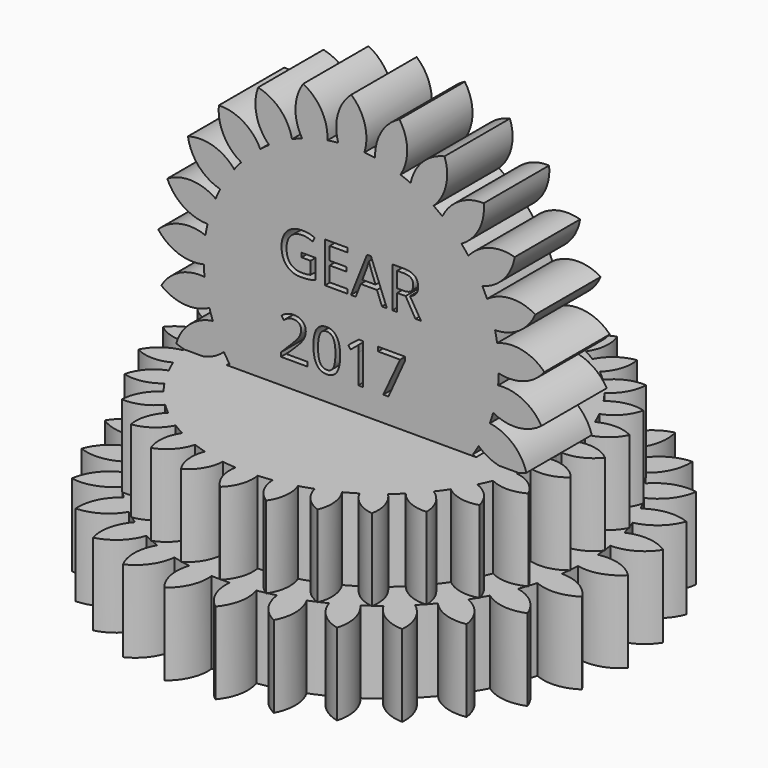
from build123d import *

# Parameters (mm, degrees)
F1_DEPTH     = 25.4
F3_DEPTH     = 25.4
F5_DEPTH     = 12.7
F6_TEXT_SIZE = 17.6388888889
F7_DEPTH     = 88.1229748473


# Not quite as in the source:
# - Text() gives the source's letters only with a copy of the font that has no kerning and outlines rounded to 1/6400 em; it was checked with that copy


with BuildPart() as f1:
    # F0 (on Top) → F1 (new body)
    with BuildSketch(Plane.XY):
        with BuildLine():
            ThreePointArc((63.3843742532, -3.8302872647), (63.4710869809, -1.9160160388), (63.5, 0))
            ThreePointArc((63.5, 0), (63.4710869809, 1.9160160388), (63.3843742532, 3.8302872647))
            ThreePointArc((63.3843742532, 3.8302872647), (63.1521403559, 6.6375574175), (62.7956351013, 9.4317661243))
            ThreePointArc((62.7956351013, 9.4317661243), (62.1123726466, 13.2023923669), (61.2029120983, 16.9249387205))
            ThreePointArc((61.2029120983, 16.9249387205), (60.3920887847, 19.6225791428), (59.4624253686, 22.2816060751))
            ThreePointArc((59.4624253686, 22.2816060751), (58.0101365603, 25.8277768353), (56.3465890005, 29.2798891393))
            ThreePointArc((56.3465890005, 29.2798891393), (54.9926131403, 31.75), (53.5304223149, 34.1576329213))
            ThreePointArc((53.5304223149, 34.1576329213), (51.3725791428, 37.3243635206), (49.0276495824, 40.3551679023))
            ThreePointArc((49.0276495824, 40.3551679023), (47.1896964178, 42.4897935038), (45.2588829386, 44.5408073024))
            ThreePointArc((45.2588829386, 44.5408073024), (42.4897935038, 47.1896964178), (39.5659666169, 49.6667321823))
            ThreePointArc((39.5659666169, 49.6667321823), (37.3243635206, 51.3725791428), (35.0093132016, 52.9773346739))
            ThreePointArc((35.0093132016, 52.9773346739), (31.75, 54.9926131403), (28.3750610516, 56.8076219386))
            ThreePointArc((28.3750610516, 56.8076219386), (25.8277768353, 58.0101365603), (23.2296684844, 59.0984983067))
            ThreePointArc((23.2296684844, 59.0984983067), (19.6225791428, 60.3920887847), (15.9440291597, 61.4657460229))
            ThreePointArc((15.9440291597, 61.4657460229), (13.2023923669, 62.1123726466), (10.4347757862, 62.6367739774))
            ThreePointArc((10.4347757862, 62.6367739774), (6.6375574175, 63.1521403559), (2.8161666856, 63.4375220607))
            ThreePointArc((2.8161666856, 63.4375220607), (0, 63.5), (-2.8161666856, 63.4375220607))
            ThreePointArc((-2.8161666856, 63.4375220607), (-6.6375574175, 63.1521403559), (-10.4347757862, 62.6367739774))
            ThreePointArc((-10.4347757862, 62.6367739774), (-13.2023923669, 62.1123726466), (-15.9440291597, 61.4657460229))
            ThreePointArc((-15.9440291597, 61.4657460229), (-19.6225791428, 60.3920887847), (-23.2296684844, 59.0984983067))
            ThreePointArc((-23.2296684844, 59.0984983067), (-25.8277768353, 58.0101365603), (-28.3750610516, 56.8076219386))
            ThreePointArc((-28.3750610516, 56.8076219386), (-31.75, 54.9926131403), (-35.0093132016, 52.9773346739))
            ThreePointArc((-35.0093132016, 52.9773346739), (-37.3243635206, 51.3725791428), (-39.5659666169, 49.6667321823))
            ThreePointArc((-39.5659666169, 49.6667321823), (-42.4897935038, 47.1896964178), (-45.2588829386, 44.5408073024))
            ThreePointArc((-45.2588829386, 44.5408073024), (-47.1896964178, 42.4897935038), (-49.0276495824, 40.3551679023))
            ThreePointArc((-49.0276495824, 40.3551679023), (-51.3725791428, 37.3243635206), (-53.5304223149, 34.1576329213))
            ThreePointArc((-53.5304223149, 34.1576329213), (-54.9926131403, 31.75), (-56.3465890005, 29.2798891393))
            ThreePointArc((-56.3465890005, 29.2798891393), (-58.0101365603, 25.8277768353), (-59.4624253686, 22.2816060751))
            ThreePointArc((-59.4624253686, 22.2816060751), (-60.3920887847, 19.6225791428), (-61.2029120983, 16.9249387205))
            ThreePointArc((-61.2029120983, 16.9249387205), (-62.1123726466, 13.2023923669), (-62.7956351013, 9.4317661243))
            ThreePointArc((-62.7956351013, 9.4317661243), (-63.1521403559, 6.6375574175), (-63.3843742532, 3.8302872647))
            ThreePointArc((-63.3843742532, 3.8302872647), (-63.5, 0), (-63.3843742532, -3.8302872647))
            ThreePointArc((-63.3843742532, -3.8302872647), (-63.1521403559, -6.6375574175), (-62.7956351013, -9.4317661243))
            ThreePointArc((-62.7956351013, -9.4317661243), (-62.1123726466, -13.2023923669), (-61.2029120983, -16.9249387205))
            ThreePointArc((-61.2029120983, -16.9249387205), (-60.3920887847, -19.6225791428), (-59.4624253686, -22.2816060751))
            ThreePointArc((-59.4624253686, -22.2816060751), (-58.0101365603, -25.8277768353), (-56.3465890005, -29.2798891393))
            ThreePointArc((-56.3465890005, -29.2798891393), (-54.9926131403, -31.75), (-53.5304223149, -34.1576329213))
            ThreePointArc((-53.5304223149, -34.1576329213), (-51.3725791428, -37.3243635206), (-49.0276495824, -40.3551679023))
            ThreePointArc((-49.0276495824, -40.3551679023), (-47.1896964178, -42.4897935038), (-45.2588829386, -44.5408073024))
            ThreePointArc((-45.2588829386, -44.5408073024), (-42.4897935038, -47.1896964178), (-39.5659666169, -49.6667321823))
            ThreePointArc((-39.5659666169, -49.6667321823), (-37.3243635206, -51.3725791428), (-35.0093132016, -52.9773346739))
            ThreePointArc((-35.0093132016, -52.9773346739), (-31.75, -54.9926131403), (-28.3750610516, -56.8076219386))
            ThreePointArc((-28.3750610516, -56.8076219386), (-25.8277768353, -58.0101365603), (-23.2296684844, -59.0984983067))
            ThreePointArc((-23.2296684844, -59.0984983067), (-19.6225791428, -60.3920887847), (-15.9440291597, -61.4657460229))
            ThreePointArc((-15.9440291597, -61.4657460229), (-13.2023923669, -62.1123726466), (-10.4347757862, -62.6367739774))
            ThreePointArc((-10.4347757862, -62.6367739774), (-6.6375574175, -63.1521403559), (-2.8161666856, -63.4375220607))
            ThreePointArc((-2.8161666856, -63.4375220607), (0, -63.5), (2.8161666856, -63.4375220607))
            ThreePointArc((2.8161666856, -63.4375220607), (6.6375574175, -63.1521403559), (10.4347757862, -62.6367739774))
            ThreePointArc((10.4347757862, -62.6367739774), (13.2023923669, -62.1123726466), (15.9440291597, -61.4657460229))
            ThreePointArc((15.9440291597, -61.4657460229), (19.6225791428, -60.3920887847), (23.2296684844, -59.0984983067))
            ThreePointArc((23.2296684844, -59.0984983067), (25.8277768353, -58.0101365603), (28.3750610516, -56.8076219386))
            ThreePointArc((28.3750610516, -56.8076219386), (31.75, -54.9926131403), (35.0093132016, -52.9773346739))
            ThreePointArc((35.0093132016, -52.9773346739), (37.3243635206, -51.3725791428), (39.5659666169, -49.6667321823))
            ThreePointArc((39.5659666169, -49.6667321823), (42.4897935038, -47.1896964178), (45.2588829386, -44.5408073024))
            ThreePointArc((45.2588829386, -44.5408073024), (47.1896964178, -42.4897935038), (49.0276495824, -40.3551679023))
            ThreePointArc((49.0276495824, -40.3551679023), (51.3725791428, -37.3243635206), (53.5304223149, -34.1576329213))
            ThreePointArc((53.5304223149, -34.1576329213), (54.9926131403, -31.75), (56.3465890005, -29.2798891393))
            ThreePointArc((56.3465890005, -29.2798891393), (58.0101365603, -25.8277768353), (59.4624253686, -22.2816060751))
            ThreePointArc((59.4624253686, -22.2816060751), (60.3920887847, -19.6225791428), (61.2029120983, -16.9249387205))
            ThreePointArc((61.2029120983, -16.9249387205), (62.1123726466, -13.2023923669), (62.7956351013, -9.4317661243))
            ThreePointArc((62.7956351013, -9.4317661243), (63.1521403559, -6.6375574175), (63.3843742532, -3.8302872647))
        make_face()
        with BuildLine():
            ThreePointArc((63.3843742532, 3.8302872647), (63.4710869809, 1.9160160388), (63.5, 0))
            ThreePointArc((63.5, 0), (63.4710869809, -1.9160160388), (63.3843742532, -3.8302872647))
            ThreePointArc((63.3843742532, -3.8302872647), (70.1108387826, -3.5405557516), (75.83742017, 0))
            ThreePointArc((75.83742017, 0), (70.1108387826, 3.5405557516), (63.3843742532, 3.8302872647))
        make_face()
        with BuildLine():
            ThreePointArc((61.2029120983, 16.9249387205), (62.1123726466, 13.2023923669), (62.7956351013, 9.4317661243))
            ThreePointArc((62.7956351013, 9.4317661243), (69.3148716734, 11.1136769223), (74.1801905851, 15.7674862548))
            ThreePointArc((74.1801905851, 15.7674862548), (67.8426258079, 18.0400491496), (61.2029120983, 16.9249387205))
        make_face()
        with BuildLine():
            ThreePointArc((74.1801905851, -15.7674862548), (69.3148716734, -11.1136769223), (62.7956351013, -9.4317661243))
            ThreePointArc((62.7956351013, -9.4317661243), (62.1123726466, -13.2023923669), (61.2029120983, -16.9249387205))
            ThreePointArc((61.2029120983, -16.9249387205), (67.8426258079, -18.0400491496), (74.1801905851, -15.7674862548))
        make_face()
        with BuildLine():
            ThreePointArc((56.3465890005, 29.2798891393), (58.0101365603, 25.8277768353), (59.4624253686, 22.2816060751))
            ThreePointArc((59.4624253686, 22.2816060751), (65.4895120624, 25.2821885853), (69.2809307156, 30.8458576995))
            ThreePointArc((69.2809307156, 30.8458576995), (62.6093645404, 31.751105834), (56.3465890005, 29.2798891393))
        make_face()
        with BuildLine():
            ThreePointArc((69.2809307156, -30.8458576995), (65.4895120624, -25.2821885853), (59.4624253686, -22.2816060751))
            ThreePointArc((59.4624253686, -22.2816060751), (58.0101365603, -25.8277768353), (56.3465890005, -29.2798891393))
            ThreePointArc((56.3465890005, -29.2798891393), (62.6093645404, -31.751105834), (69.2809307156, -30.8458576995))
        make_face()
        with BuildLine():
            ThreePointArc((49.0276495824, 40.3551679023), (51.3725791428, 37.3243635206), (53.5304223149, 34.1576329213))
            ThreePointArc((53.5304223149, 34.1576329213), (58.8019465207, 38.3457472898), (61.3537617271, 44.5761171478))
            ThreePointArc((61.3537617271, 44.5761171478), (54.6397736094, 44.0744868348), (49.0276495824, 40.3551679023))
        make_face()
        with BuildLine():
            ThreePointArc((61.3537617271, -44.5761171478), (58.8019465207, -38.3457472898), (53.5304223149, -34.1576329213))
            ThreePointArc((53.5304223149, -34.1576329213), (51.3725791428, -37.3243635206), (49.0276495824, -40.3551679023))
            ThreePointArc((49.0276495824, -40.3551679023), (54.6397736094, -44.0744868348), (61.3537617271, -44.5761171478))
        make_face()
        with BuildLine():
            ThreePointArc((39.5659666169, 49.6667321823), (42.4897935038, 47.1896964178), (45.2588829386, 44.5408073024))
            ThreePointArc((45.2588829386, 44.5408073024), (49.544453753, 49.7334128343), (50.745138943, 56.3581863769))
            ThreePointArc((50.745138943, 56.3581863769), (44.2821623809, 54.4716012681), (39.5659666169, 49.6667321823))
        make_face()
        with BuildLine():
            ThreePointArc((50.745138943, -56.3581863769), (49.544453753, -49.7334128343), (45.2588829386, -44.5408073024))
            ThreePointArc((45.2588829386, -44.5408073024), (42.4897935038, -47.1896964178), (39.5659666169, -49.6667321823))
            ThreePointArc((39.5659666169, -49.6667321823), (44.2821623809, -54.4716012681), (50.745138943, -56.3581863769))
        make_face()
        with BuildLine():
            ThreePointArc((28.3750610516, 56.8076219386), (31.75, 54.9926131403), (35.0093132016, 52.9773346739))
            ThreePointArc((35.0093132016, 52.9773346739), (38.1216306157, 58.9474895906), (37.918710085, 65.6771324247))
            ThreePointArc((37.918710085, 65.6771324247), (31.989208167, 62.4880453422), (28.3750610516, 56.8076219386))
        make_face()
        with BuildLine():
            ThreePointArc((37.918710085, -65.6771324247), (38.1216306157, -58.9474895906), (35.0093132016, -52.9773346739))
            ThreePointArc((35.0093132016, -52.9773346739), (31.75, -54.9926131403), (28.3750610516, -56.8076219386))
            ThreePointArc((28.3750610516, -56.8076219386), (31.989208167, -62.4880453422), (37.918710085, -65.6771324247))
        make_face()
        with BuildLine():
            ThreePointArc((15.9440291597, 61.4657460229), (19.6225791428, 60.3920887847), (23.2296684844, 59.0984983067))
            ThreePointArc((23.2296684844, 59.0984983067), (25.0327092925, 65.5852781904), (23.4350516421, 72.1256726317))
            ThreePointArc((23.4350516421, 72.1256726317), (18.2981720549, 67.7734619839), (15.9440291597, 61.4657460229))
        make_face()
        with BuildLine():
            ThreePointArc((23.4350516421, -72.1256726317), (25.0327092925, -65.5852781904), (23.2296684844, -59.0984983067))
            ThreePointArc((23.2296684844, -59.0984983067), (19.6225791428, -60.3920887847), (15.9440291597, -61.4657460229))
            ThreePointArc((15.9440291597, -61.4657460229), (18.2981720549, -67.7734619839), (23.4350516421, -72.1256726317))
        make_face()
        with BuildLine():
            ThreePointArc((2.8161666856, 63.4375220607), (6.6375574175, 63.1521403559), (10.4347757862, 62.6367739774))
            ThreePointArc((10.4347757862, 62.6367739774), (10.849738453, 69.3566754201), (7.9271689885, 75.4219748473))
            ThreePointArc((7.9271689885, 75.4219748473), (3.8074180197, 70.0968531238), (2.8161666856, 63.4375220607))
        make_face()
        with BuildLine():
            ThreePointArc((7.9271689885, -75.4219748473), (10.849738453, -69.3566754201), (10.4347757862, -62.6367739774))
            ThreePointArc((10.4347757862, -62.6367739774), (6.6375574175, -63.1521403559), (2.8161666856, -63.4375220607))
            ThreePointArc((2.8161666856, -63.4375220607), (3.8074180197, -70.0968531238), (7.9271689885, -75.4219748473))
        make_face()
        with BuildLine():
            ThreePointArc((-10.4347757862, 62.6367739774), (-6.6375574175, 63.1521403559), (-2.8161666856, 63.4375220607))
            ThreePointArc((-2.8161666856, 63.4375220607), (-3.8074180197, 70.0968531238), (-7.9271689885, 75.4219748473))
            ThreePointArc((-7.9271689885, 75.4219748473), (-10.849738453, 69.3566754201), (-10.4347757862, 62.6367739774))
        make_face()
        with BuildLine():
            ThreePointArc((-7.9271689885, -75.4219748473), (-3.8074180197, -70.0968531238), (-2.8161666856, -63.4375220607))
            ThreePointArc((-2.8161666856, -63.4375220607), (-6.6375574175, -63.1521403559), (-10.4347757862, -62.6367739774))
            ThreePointArc((-10.4347757862, -62.6367739774), (-10.849738453, -69.3566754201), (-7.9271689885, -75.4219748473))
        make_face()
        with BuildLine():
            ThreePointArc((-23.2296684844, 59.0984983067), (-19.6225791428, 60.3920887847), (-15.9440291597, 61.4657460229))
            ThreePointArc((-15.9440291597, 61.4657460229), (-18.2981720549, 67.7734619839), (-23.4350516421, 72.1256726317))
            ThreePointArc((-23.4350516421, 72.1256726317), (-25.0327092925, 65.5852781904), (-23.2296684844, 59.0984983067))
        make_face()
        with BuildLine():
            ThreePointArc((-23.4350516421, -72.1256726317), (-18.2981720549, -67.7734619839), (-15.9440291597, -61.4657460229))
            ThreePointArc((-15.9440291597, -61.4657460229), (-19.6225791428, -60.3920887847), (-23.2296684844, -59.0984983067))
            ThreePointArc((-23.2296684844, -59.0984983067), (-25.0327092925, -65.5852781904), (-23.4350516421, -72.1256726317))
        make_face()
        with BuildLine():
            ThreePointArc((-35.0093132016, 52.9773346739), (-31.75, 54.9926131403), (-28.3750610516, 56.8076219386))
            ThreePointArc((-28.3750610516, 56.8076219386), (-31.989208167, 62.4880453422), (-37.918710085, 65.6771324247))
            ThreePointArc((-37.918710085, 65.6771324247), (-38.1216306157, 58.9474895906), (-35.0093132016, 52.9773346739))
        make_face()
        with BuildLine():
            ThreePointArc((-37.918710085, -65.6771324247), (-31.989208167, -62.4880453422), (-28.3750610516, -56.8076219386))
            ThreePointArc((-28.3750610516, -56.8076219386), (-31.75, -54.9926131403), (-35.0093132016, -52.9773346739))
            ThreePointArc((-35.0093132016, -52.9773346739), (-38.1216306157, -58.9474895906), (-37.918710085, -65.6771324247))
        make_face()
        with BuildLine():
            ThreePointArc((-45.2588829386, 44.5408073024), (-42.4897935038, 47.1896964178), (-39.5659666169, 49.6667321823))
            ThreePointArc((-39.5659666169, 49.6667321823), (-44.2821623809, 54.4716012681), (-50.745138943, 56.3581863769))
            ThreePointArc((-50.745138943, 56.3581863769), (-49.544453753, 49.7334128343), (-45.2588829386, 44.5408073024))
        make_face()
        with BuildLine():
            ThreePointArc((-50.745138943, -56.3581863769), (-44.2821623809, -54.4716012681), (-39.5659666169, -49.6667321823))
            ThreePointArc((-39.5659666169, -49.6667321823), (-42.4897935038, -47.1896964178), (-45.2588829386, -44.5408073024))
            ThreePointArc((-45.2588829386, -44.5408073024), (-49.544453753, -49.7334128343), (-50.745138943, -56.3581863769))
        make_face()
        with BuildLine():
            ThreePointArc((-53.5304223149, 34.1576329213), (-51.3725791428, 37.3243635206), (-49.0276495824, 40.3551679023))
            ThreePointArc((-49.0276495824, 40.3551679023), (-54.6397736094, 44.0744868348), (-61.3537617271, 44.5761171478))
            ThreePointArc((-61.3537617271, 44.5761171478), (-58.8019465207, 38.3457472898), (-53.5304223149, 34.1576329213))
        make_face()
        with BuildLine():
            ThreePointArc((-61.3537617271, -44.5761171478), (-54.6397736094, -44.0744868348), (-49.0276495824, -40.3551679023))
            ThreePointArc((-49.0276495824, -40.3551679023), (-51.3725791428, -37.3243635206), (-53.5304223149, -34.1576329213))
            ThreePointArc((-53.5304223149, -34.1576329213), (-58.8019465207, -38.3457472898), (-61.3537617271, -44.5761171478))
        make_face()
        with BuildLine():
            ThreePointArc((-59.4624253686, 22.2816060751), (-58.0101365603, 25.8277768353), (-56.3465890005, 29.2798891393))
            ThreePointArc((-56.3465890005, 29.2798891393), (-62.6093645404, 31.751105834), (-69.2809307156, 30.8458576995))
            ThreePointArc((-69.2809307156, 30.8458576995), (-65.4895120624, 25.2821885853), (-59.4624253686, 22.2816060751))
        make_face()
        with BuildLine():
            ThreePointArc((-69.2809307156, -30.8458576995), (-62.6093645404, -31.751105834), (-56.3465890005, -29.2798891393))
            ThreePointArc((-56.3465890005, -29.2798891393), (-58.0101365603, -25.8277768353), (-59.4624253686, -22.2816060751))
            ThreePointArc((-59.4624253686, -22.2816060751), (-65.4895120624, -25.2821885853), (-69.2809307156, -30.8458576995))
        make_face()
        with BuildLine():
            ThreePointArc((-62.7956351013, 9.4317661243), (-62.1123726466, 13.2023923669), (-61.2029120983, 16.9249387205))
            ThreePointArc((-61.2029120983, 16.9249387205), (-67.8426258079, 18.0400491496), (-74.1801905851, 15.7674862548))
            ThreePointArc((-74.1801905851, 15.7674862548), (-69.3148716734, 11.1136769223), (-62.7956351013, 9.4317661243))
        make_face()
        with BuildLine():
            ThreePointArc((-74.1801905851, -15.7674862548), (-67.8426258079, -18.0400491496), (-61.2029120983, -16.9249387205))
            ThreePointArc((-61.2029120983, -16.9249387205), (-62.1123726466, -13.2023923669), (-62.7956351013, -9.4317661243))
            ThreePointArc((-62.7956351013, -9.4317661243), (-69.3148716734, -11.1136769223), (-74.1801905851, -15.7674862548))
        make_face()
        with BuildLine():
            ThreePointArc((-63.3843742532, -3.8302872647), (-63.9551391112, 0), (-63.3843742532, 3.8302872647))
            ThreePointArc((-63.3843742532, 3.8302872647), (-70.1108387826, 3.5405557516), (-75.83742017, 0))
            ThreePointArc((-75.83742017, 0), (-70.1108387826, -3.5405557516), (-63.3843742532, -3.8302872647))
        make_face()
        with BuildLine():
            ThreePointArc((-63.3843742532, -3.8302872647), (-63.5, 0), (-63.3843742532, 3.8302872647))
            ThreePointArc((-63.3843742532, 3.8302872647), (-63.9551391112, 0), (-63.3843742532, -3.8302872647))
        make_face()
    extrude(amount=F1_DEPTH)

    # F2 (on face) → F3 (join)
    with BuildSketch(Plane.XY.offset(25.4)):
        with BuildLine():
            ThreePointArc((53.4574080141, -2.1584102312), (53.4900742973, -1.0794248349), (53.5009645362, 0))
            ThreePointArc((53.5009645362, 0), (53.4900742973, 1.0794248349), (53.4574080141, 2.1584102312))
            ThreePointArc((53.4574080141, 2.1584102312), (53.2078806546, 5.5923736063), (52.7379941111, 9.0031762979))
            ThreePointArc((52.7379941111, 9.0031762979), (52.3318400981, 11.1234759971), (51.8404766698, 13.225663876))
            ThreePointArc((51.8404766698, 13.225663876), (50.8824409503, 16.5327072572), (49.7136768004, 19.7712808207))
            ThreePointArc((49.7136768004, 19.7712808207), (48.8755631316, 21.7608027168), (47.9578677368, 23.7148925456))
            ThreePointArc((47.9578677368, 23.7148925456), (46.3331944154, 26.7504822681), (44.5166332609, 29.6752854986))
            ThreePointArc((44.5166332609, 29.6752854986), (43.2831895253, 31.4470779378), (41.9792698563, 33.1676666143))
            ThreePointArc((41.9792698563, 33.1676666143), (39.7589649532, 35.7991328409), (37.3739992334, 38.2823378023))
            ThreePointArc((37.3739992334, 38.2823378023), (35.7991328409, 39.7589649532), (34.1659764442, 41.1708544959))
            ThreePointArc((34.1659764442, 41.1708544959), (31.4470779378, 43.2831895253), (28.5979420991, 45.216268245))
            ThreePointArc((28.5979420991, 45.216268245), (26.7504822681, 46.3331944154), (24.859465915, 47.3746784763))
            ThreePointArc((24.859465915, 47.3746784763), (21.7608027168, 48.8755631316), (18.5720176668, 50.1740307937))
            ThreePointArc((18.5720176668, 50.1740307937), (16.5327072572, 50.8824409503), (14.4664774363, 51.5080016783))
            ThreePointArc((14.4664774363, 51.5080016783), (11.1234759971, 52.3318400981), (7.7344069441, 52.9389474351))
            ThreePointArc((7.7344069441, 52.9389474351), (5.5923736063, 53.2078806546), (3.4412344758, 53.3901780442))
            ThreePointArc((3.4412344758, 53.3901780442), (0, 53.5009645362), (-3.4412344758, 53.3901780442))
            ThreePointArc((-3.4412344758, 53.3901780442), (-5.5923736063, 53.2078806546), (-7.7344069441, 52.9389474351))
            ThreePointArc((-7.7344069441, 52.9389474351), (-11.1234759971, 52.3318400981), (-14.4664774363, 51.5080016783))
            ThreePointArc((-14.4664774363, 51.5080016783), (-16.5327072572, 50.8824409503), (-18.5720176668, 50.1740307937))
            ThreePointArc((-18.5720176668, 50.1740307937), (-21.7608027168, 48.8755631316), (-24.859465915, 47.3746784763))
            ThreePointArc((-24.859465915, 47.3746784763), (-26.7504822681, 46.3331944154), (-28.5979420991, 45.216268245))
            ThreePointArc((-28.5979420991, 45.216268245), (-31.4470779378, 43.2831895253), (-34.1659764442, 41.1708544959))
            ThreePointArc((-34.1659764442, 41.1708544959), (-35.7991328409, 39.7589649532), (-37.3739992334, 38.2823378023))
            ThreePointArc((-37.3739992334, 38.2823378023), (-39.7589649532, 35.7991328409), (-41.9792698563, 33.1676666143))
            ThreePointArc((-41.9792698563, 33.1676666143), (-43.2831895253, 31.4470779378), (-44.5166332609, 29.6752854986))
            ThreePointArc((-44.5166332609, 29.6752854986), (-46.3331944154, 26.7504822681), (-47.9578677368, 23.7148925456))
            ThreePointArc((-47.9578677368, 23.7148925456), (-48.8755631316, 21.7608027168), (-49.7136768004, 19.7712808207))
            ThreePointArc((-49.7136768004, 19.7712808207), (-50.8824409503, 16.5327072572), (-51.8404766698, 13.225663876))
            ThreePointArc((-51.8404766698, 13.225663876), (-52.3318400981, 11.1234759971), (-52.7379941111, 9.0031762979))
            ThreePointArc((-52.7379941111, 9.0031762979), (-52.9098679132, 7.2911544424), (-53.0870626478, 5.5796751221))
            ThreePointArc((-53.0870626478, 5.5796751221), (-53.2695766026, 3.8687548744), (-53.4574080141, 2.1584102312))
            ThreePointArc((-53.4574080141, 2.1584102312), (-53.5009645362, 0), (-53.4574080141, -2.1584102312))
            ThreePointArc((-53.4574080141, -2.1584102312), (-53.2078806546, -5.5923736063), (-52.7379941111, -9.0031762979))
            ThreePointArc((-52.7379941111, -9.0031762979), (-52.3318400981, -11.1234759971), (-51.8404766698, -13.225663876))
            ThreePointArc((-51.8404766698, -13.225663876), (-50.8824409503, -16.5327072572), (-49.7136768004, -19.7712808207))
            ThreePointArc((-49.7136768004, -19.7712808207), (-48.8755631316, -21.7608027168), (-47.9578677368, -23.7148925456))
            ThreePointArc((-47.9578677368, -23.7148925456), (-46.3331944154, -26.7504822681), (-44.5166332609, -29.6752854986))
            ThreePointArc((-44.5166332609, -29.6752854986), (-43.2831895253, -31.4470779378), (-41.9792698563, -33.1676666143))
            ThreePointArc((-41.9792698563, -33.1676666143), (-39.7589649532, -35.7991328409), (-37.3739992334, -38.2823378023))
            ThreePointArc((-37.3739992334, -38.2823378023), (-35.7991328409, -39.7589649532), (-34.1659764442, -41.1708544959))
            ThreePointArc((-34.1659764442, -41.1708544959), (-31.4470779378, -43.2831895253), (-28.5979420991, -45.216268245))
            ThreePointArc((-28.5979420991, -45.216268245), (-26.7504822681, -46.3331944154), (-24.859465915, -47.3746784763))
            ThreePointArc((-24.859465915, -47.3746784763), (-21.7608027168, -48.8755631316), (-18.5720176668, -50.1740307937))
            ThreePointArc((-18.5720176668, -50.1740307937), (-16.5327072572, -50.8824409503), (-14.4664774363, -51.5080016783))
            ThreePointArc((-14.4664774363, -51.5080016783), (-11.1234759971, -52.3318400981), (-7.7344069441, -52.9389474351))
            ThreePointArc((-7.7344069441, -52.9389474351), (-5.5923736063, -53.2078806546), (-3.4412344758, -53.3901780442))
            ThreePointArc((-3.4412344758, -53.3901780442), (0, -53.5009645362), (3.4412344758, -53.3901780442))
            ThreePointArc((3.4412344758, -53.3901780442), (5.5923736063, -53.2078806546), (7.7344069441, -52.9389474351))
            ThreePointArc((7.7344069441, -52.9389474351), (11.1234759971, -52.3318400981), (14.4664774363, -51.5080016783))
            ThreePointArc((14.4664774363, -51.5080016783), (16.5327072572, -50.8824409503), (18.5720176668, -50.1740307937))
            ThreePointArc((18.5720176668, -50.1740307937), (21.7608027168, -48.8755631316), (24.859465915, -47.3746784763))
            ThreePointArc((24.859465915, -47.3746784763), (26.7504822681, -46.3331944154), (28.5979420991, -45.216268245))
            ThreePointArc((28.5979420991, -45.216268245), (31.4470779378, -43.2831895253), (34.1659764442, -41.1708544959))
            ThreePointArc((34.1659764442, -41.1708544959), (35.7991328409, -39.7589649532), (37.3739992334, -38.2823378023))
            ThreePointArc((37.3739992334, -38.2823378023), (39.7589649532, -35.7991328409), (41.9792698563, -33.1676666143))
            ThreePointArc((41.9792698563, -33.1676666143), (43.2831895253, -31.4470779378), (44.5166332609, -29.6752854986))
            ThreePointArc((44.5166332609, -29.6752854986), (46.3331944154, -26.7504822681), (47.9578677368, -23.7148925456))
            ThreePointArc((47.9578677368, -23.7148925456), (48.8755631316, -21.7608027168), (49.7136768004, -19.7712808207))
            ThreePointArc((49.7136768004, -19.7712808207), (50.8824409503, -16.5327072572), (51.8404766698, -13.225663876))
            ThreePointArc((51.8404766698, -13.225663876), (52.3318400981, -11.1234759971), (52.7379941111, -9.0031762979))
            ThreePointArc((52.7379941111, -9.0031762979), (53.2078806546, -5.5923736063), (53.4574080141, -2.1584102312))
        make_face()
        with BuildLine():
            ThreePointArc((52.7379941111, 9.0031762979), (53.2078806546, 5.5923736063), (53.4574080141, 2.1584102312))
            ThreePointArc((53.4574080141, 2.1584102312), (58.9731507298, 3.1661170371), (63.3590941473, 6.6593091375))
            ThreePointArc((63.3590941473, 6.6593091375), (58.3427186405, 9.1642776976), (52.7379941111, 9.0031762979))
        make_face()
        with BuildLine():
            ThreePointArc((63.3590941473, -6.6593091375), (58.9731507298, -3.1661170371), (53.4574080141, -2.1584102312))
            ThreePointArc((53.4574080141, -2.1584102312), (53.2078806546, -5.5923736063), (52.7379941111, -9.0031762979))
            ThreePointArc((52.7379941111, -9.0031762979), (58.3427186405, -9.1642776976), (63.3590941473, -6.6593091375))
        make_face()
        with BuildLine():
            ThreePointArc((49.7136768004, 19.7712808207), (50.8824409503, 16.5327072572), (51.8404766698, 13.225663876))
            ThreePointArc((51.8404766698, 13.225663876), (57.0261731475, 15.3581372645), (60.5899977024, 19.6868836482))
            ThreePointArc((60.5899977024, 19.6868836482), (55.1624297873, 21.0941495218), (49.7136768004, 19.7712808207))
        make_face()
        with BuildLine():
            ThreePointArc((60.5899977024, -19.6868836482), (57.0261731475, -15.3581372645), (51.8404766698, -13.225663876))
            ThreePointArc((51.8404766698, -13.225663876), (50.8824409503, -16.5327072572), (49.7136768004, -19.7712808207))
            ThreePointArc((49.7136768004, -19.7712808207), (55.1624297873, -21.0941495218), (60.5899977024, -19.6868836482))
        make_face()
        with BuildLine():
            ThreePointArc((44.5166332609, 29.6752854986), (46.3331944154, 26.7504822681), (47.9578677368, 23.7148925456))
            ThreePointArc((47.9578677368, 23.7148925456), (52.5868781568, 26.878933197), (55.1728276148, 31.8540468754))
            ThreePointArc((55.1728276148, 31.8540468754), (49.5712780536, 32.102105791), (44.5166332609, 29.6752854986))
        make_face()
        with BuildLine():
            ThreePointArc((55.1728276148, -31.8540468754), (52.5868781568, -26.878933197), (47.9578677368, -23.7148925456))
            ThreePointArc((47.9578677368, -23.7148925456), (46.3331944154, -26.7504822681), (44.5166332609, -29.6752854986))
            ThreePointArc((44.5166332609, -29.6752854986), (49.5712780536, -32.102105791), (55.1728276148, -31.8540468754))
        make_face()
        with BuildLine():
            ThreePointArc((37.3739992334, 38.2823378023), (39.7589649532, 35.7991328409), (41.9792698563, 33.1676666143))
            ThreePointArc((41.9792698563, 33.1676666143), (45.8492842508, 37.2249907694), (47.3443402119, 42.6290354014))
            ThreePointArc((47.3443402119, 42.6290354014), (41.8136235997, 41.7070459941), (37.3739992334, 38.2823378023))
        make_face()
        with BuildLine():
            ThreePointArc((47.3443402119, -42.6290354014), (45.8492842508, -37.2249907694), (41.9792698563, -33.1676666143))
            ThreePointArc((41.9792698563, -33.1676666143), (39.7589649532, -35.7991328409), (37.3739992334, -38.2823378023))
            ThreePointArc((37.3739992334, -38.2823378023), (41.8136235997, -41.7070459941), (47.3443402119, -42.6290354014))
        make_face()
        with BuildLine():
            ThreePointArc((28.5979420991, 45.216268245), (31.4470779378, 43.2831895253), (34.1659764442, 41.1708544959))
            ThreePointArc((34.1659764442, 41.1708544959), (37.1078566137, 45.9441376197), (37.4466779584, 51.5409305236))
            ThreePointArc((37.4466779584, 51.5409305236), (32.2285131503, 49.4891881546), (28.5979420991, 45.216268245))
        make_face()
        with BuildLine():
            ThreePointArc((37.4466779584, -51.5409305236), (37.1078566137, -45.9441376197), (34.1659764442, -41.1708544959))
            ThreePointArc((34.1659764442, -41.1708544959), (31.4470779378, -43.2831895253), (28.5979420991, -45.216268245))
            ThreePointArc((28.5979420991, -45.216268245), (32.2285131503, -49.4891881546), (37.4466779584, -51.5409305236))
        make_face()
        with BuildLine():
            ThreePointArc((18.5720176668, 50.1740307937), (21.7608027168, 48.8755631316), (24.859465915, 47.3746784763))
            ThreePointArc((24.859465915, 47.3746784763), (26.7446375794, 52.6553051917), (25.9124161889, 58.2002396611))
            ThreePointArc((25.9124161889, 58.2002396611), (21.2348620268, 55.1084153173), (18.5720176668, 50.1740307937))
        make_face()
        with BuildLine():
            ThreePointArc((25.9124161889, -58.2002396611), (26.7446375794, -52.6553051917), (24.859465915, -47.3746784763))
            ThreePointArc((24.859465915, -47.3746784763), (21.7608027168, -48.8755631316), (18.5720176668, -50.1740307937))
            ThreePointArc((18.5720176668, -50.1740307937), (21.2348620268, -55.1084153173), (25.9124161889, -58.2002396611))
        make_face()
        with BuildLine():
            ThreePointArc((7.7344069441, 52.9389474351), (11.1234759971, 52.3318400981), (14.4664774363, 51.5080016783))
            ThreePointArc((14.4664774363, 51.5080016783), (15.2125495479, 57.0651832586), (13.2456574905, 62.3159190496))
            ThreePointArc((13.2456574905, 62.3159190496), (9.3131455365, 58.3191402912), (7.7344069441, 52.9389474351))
        make_face()
        with BuildLine():
            ThreePointArc((13.2456574905, -62.3159190496), (15.2125495479, -57.0651832586), (14.4664774363, -51.5080016783))
            ThreePointArc((14.4664774363, -51.5080016783), (11.1234759971, -52.3318400981), (7.7344069441, -52.9389474351))
            ThreePointArc((7.7344069441, -52.9389474351), (9.3131455365, -58.3191402912), (13.2456574905, -62.3159190496))
        make_face()
        with BuildLine():
            ThreePointArc((-3.4412344758, 53.3901780442), (0, 53.5009645362), (3.4412344758, 53.3901780442))
            ThreePointArc((3.4412344758, 53.3901780442), (3.0156001031, 58.981038988), (0, 63.7080937508))
            ThreePointArc((0, 63.7080937508), (-3.0156001031, 58.981038988), (-3.4412344758, 53.3901780442))
        make_face()
        with BuildLine():
            ThreePointArc((0, -63.7080937508), (3.0156001031, -58.981038988), (3.4412344758, -53.3901780442))
            ThreePointArc((3.4412344758, -53.3901780442), (0, -53.5009645362), (-3.4412344758, -53.3901780442))
            ThreePointArc((-3.4412344758, -53.3901780442), (-3.0156001031, -58.981038988), (0, -63.7080937508))
        make_face()
        with BuildLine():
            ThreePointArc((-14.4664774363, 51.5080016783), (-11.1234759971, 52.3318400981), (-7.7344069441, 52.9389474351))
            ThreePointArc((-7.7344069441, 52.9389474351), (-9.3131455365, 58.3191402912), (-13.2456574905, 62.3159190496))
            ThreePointArc((-13.2456574905, 62.3159190496), (-15.2125495479, 57.0651832586), (-14.4664774363, 51.5080016783))
        make_face()
        with BuildLine():
            ThreePointArc((-13.2456574905, -62.3159190496), (-9.3131455365, -58.3191402912), (-7.7344069441, -52.9389474351))
            ThreePointArc((-7.7344069441, -52.9389474351), (-11.1234759971, -52.3318400981), (-14.4664774363, -51.5080016783))
            ThreePointArc((-14.4664774363, -51.5080016783), (-15.2125495479, -57.0651832586), (-13.2456574905, -62.3159190496))
        make_face()
        with BuildLine():
            ThreePointArc((-24.859465915, 47.3746784763), (-21.7608027168, 48.8755631316), (-18.5720176668, 50.1740307937))
            ThreePointArc((-18.5720176668, 50.1740307937), (-21.2348620268, 55.1084153173), (-25.9124161889, 58.2002396611))
            ThreePointArc((-25.9124161889, 58.2002396611), (-26.7446375794, 52.6553051917), (-24.859465915, 47.3746784763))
        make_face()
        with BuildLine():
            ThreePointArc((-25.9124161889, -58.2002396611), (-21.2348620268, -55.1084153173), (-18.5720176668, -50.1740307937))
            ThreePointArc((-18.5720176668, -50.1740307937), (-21.7608027168, -48.8755631316), (-24.859465915, -47.3746784763))
            ThreePointArc((-24.859465915, -47.3746784763), (-26.7446375794, -52.6553051917), (-25.9124161889, -58.2002396611))
        make_face()
        with BuildLine():
            ThreePointArc((-34.1659764442, 41.1708544959), (-31.4470779378, 43.2831895253), (-28.5979420991, 45.216268245))
            ThreePointArc((-28.5979420991, 45.216268245), (-32.2285131503, 49.4891881546), (-37.4466779584, 51.5409305236))
            ThreePointArc((-37.4466779584, 51.5409305236), (-37.1078566137, 45.9441376197), (-34.1659764442, 41.1708544959))
        make_face()
        with BuildLine():
            ThreePointArc((-37.4466779584, -51.5409305236), (-32.2285131503, -49.4891881546), (-28.5979420991, -45.216268245))
            ThreePointArc((-28.5979420991, -45.216268245), (-31.4470779378, -43.2831895253), (-34.1659764442, -41.1708544959))
            ThreePointArc((-34.1659764442, -41.1708544959), (-37.1078566137, -45.9441376197), (-37.4466779584, -51.5409305236))
        make_face()
        with BuildLine():
            ThreePointArc((-41.9792698563, 33.1676666143), (-39.7589649532, 35.7991328409), (-37.3739992334, 38.2823378023))
            ThreePointArc((-37.3739992334, 38.2823378023), (-41.8136235997, 41.7070459941), (-47.3443402119, 42.6290354014))
            ThreePointArc((-47.3443402119, 42.6290354014), (-45.8492842508, 37.2249907694), (-41.9792698563, 33.1676666143))
        make_face()
        with BuildLine():
            ThreePointArc((-47.3443402119, -42.6290354014), (-41.8136235997, -41.7070459941), (-37.3739992334, -38.2823378023))
            ThreePointArc((-37.3739992334, -38.2823378023), (-39.7589649532, -35.7991328409), (-41.9792698563, -33.1676666143))
            ThreePointArc((-41.9792698563, -33.1676666143), (-45.8492842508, -37.2249907694), (-47.3443402119, -42.6290354014))
        make_face()
        with BuildLine():
            ThreePointArc((-47.9578677368, 23.7148925456), (-46.3331944154, 26.7504822681), (-44.5166332609, 29.6752854986))
            ThreePointArc((-44.5166332609, 29.6752854986), (-49.5712780536, 32.102105791), (-55.1728276148, 31.8540468754))
            ThreePointArc((-55.1728276148, 31.8540468754), (-52.5868781568, 26.878933197), (-47.9578677368, 23.7148925456))
        make_face()
        with BuildLine():
            ThreePointArc((-55.1728276148, -31.8540468754), (-49.5712780536, -32.102105791), (-44.5166332609, -29.6752854986))
            ThreePointArc((-44.5166332609, -29.6752854986), (-46.3331944154, -26.7504822681), (-47.9578677368, -23.7148925456))
            ThreePointArc((-47.9578677368, -23.7148925456), (-52.5868781568, -26.878933197), (-55.1728276148, -31.8540468754))
        make_face()
        with BuildLine():
            ThreePointArc((-51.8404766698, 13.225663876), (-50.8824409503, 16.5327072572), (-49.7136768004, 19.7712808207))
            ThreePointArc((-49.7136768004, 19.7712808207), (-55.1624297873, 21.0941495218), (-60.5899977024, 19.6868836482))
            ThreePointArc((-60.5899977024, 19.6868836482), (-57.0261731475, 15.3581372645), (-51.8404766698, 13.225663876))
        make_face()
        with BuildLine():
            ThreePointArc((-60.5899977024, -19.6868836482), (-55.1624297873, -21.0941495218), (-49.7136768004, -19.7712808207))
            ThreePointArc((-49.7136768004, -19.7712808207), (-50.8824409503, -16.5327072572), (-51.8404766698, -13.225663876))
            ThreePointArc((-51.8404766698, -13.225663876), (-57.0261731475, -15.3581372645), (-60.5899977024, -19.6868836482))
        make_face()
        with BuildLine():
            ThreePointArc((-53.0870626478, 5.5796751221), (-52.9098679132, 7.2911544424), (-52.7379941111, 9.0031762979))
            ThreePointArc((-52.7379941111, 9.0031762979), (-53.0003819676, 7.3015558337), (-53.2078806546, 5.5923736063))
            Line((-53.2078806546, 5.5923736063), (-53.0870626478, 5.5796751221))
        make_face()
        with BuildLine():
            ThreePointArc((-53.2078806546, 5.5923736063), (-53.0003819676, 7.3015558337), (-52.7379941111, 9.0031762979))
            ThreePointArc((-52.7379941111, 9.0031762979), (-58.3427186405, 9.1642776976), (-63.3590941473, 6.6593091375))
            ThreePointArc((-63.3590941473, 6.6593091375), (-58.9731507298, 3.1661170371), (-53.4574080141, 2.1584102312))
            ThreePointArc((-53.4574080141, 2.1584102312), (-53.3602752786, 3.8773997085), (-53.2078806546, 5.5923736063))
        make_face()
        with BuildLine():
            ThreePointArc((-63.3590941473, -6.6593091375), (-58.3427186405, -9.1642776976), (-52.7379941111, -9.0031762979))
            ThreePointArc((-52.7379941111, -9.0031762979), (-53.2078806546, -5.5923736063), (-53.4574080141, -2.1584102312))
            ThreePointArc((-53.4574080141, -2.1584102312), (-58.9731507298, -3.1661170371), (-63.3590941473, -6.6593091375))
        make_face()
        with BuildLine():
            Line((-53.0870626478, 5.5796751221), (-53.2078806546, 5.5923736063))
            ThreePointArc((-53.2078806546, 5.5923736063), (-53.3602752786, 3.8773997085), (-53.4574080141, 2.1584102312))
            ThreePointArc((-53.4574080141, 2.1584102312), (-53.2695766026, 3.8687548744), (-53.0870626478, 5.5796751221))
        make_face()
    extrude(amount=F3_DEPTH)

    # F4 (on Front) → F5 (join, symmetric)
    with BuildSketch(Plane.XZ):
        with BuildLine():
            ThreePointArc((45.8317549389, 76.044509612), (45.8433671556, 76.640169339), (45.8472381123, 77.2359296679))
            ThreePointArc((45.8472381123, 77.2359296679), (45.7154976418, 80.7090432407), (45.3210333338, 84.1621970673))
            ThreePointArc((45.3210333338, 84.1621970673), (45.0351574789, 85.8268454156), (44.6881601981, 87.4798342282))
            ThreePointArc((44.6881601981, 87.4798342282), (43.6033145609, 91.4035053898), (42.174697074, 95.2154783064))
            ThreePointArc((42.174697074, 95.2154783064), (41.4838213249, 96.7567342316), (40.7366440004, 98.2714966465))
            ThreePointArc((40.7366440004, 98.2714966465), (38.7101034454, 101.8021083243), (36.3783694894, 105.1390383804))
            ThreePointArc((36.3783694894, 105.1390383804), (35.3259041102, 106.4600591045), (34.2254946414, 107.7414170281))
            ThreePointArc((34.2254946414, 107.7414170281), (31.3845941646, 110.6571279058), (28.2962551595, 113.3093435136))
            ThreePointArc((28.2962551595, 113.3093435136), (26.9483304208, 114.327124446), (25.5638315814, 115.2945654476))
            ThreePointArc((25.5638315814, 115.2945654476), (22.087075408, 117.4121706873), (18.4361830516, 119.213023386))
            ThreePointArc((18.4361830516, 119.213023386), (16.8774940219, 119.8636136077), (15.295898966, 120.4563498111))
            ThreePointArc((15.295898966, 120.4563498111), (11.401744473, 121.6427924878), (7.417697759, 122.4791280793))
            ThreePointArc((7.417697759, 122.4791280793), (5.7461826026, 122.7216486139), (4.0668687642, 122.9024362234))
            ThreePointArc((4.0668687642, 122.9024362234), (0, 122.8766981927), (-4.0668687642, 122.9024362234))
            ThreePointArc((-4.0668687642, 122.9024362234), (-5.7461826026, 122.7216486139), (-7.417697759, 122.4791280793))
            ThreePointArc((-7.417697759, 122.4791280793), (-11.401744473, 121.6427924878), (-15.295898966, 120.4563498111))
            ThreePointArc((-15.295898966, 120.4563498111), (-16.8774940219, 119.8636136077), (-18.4361830516, 119.213023386))
            ThreePointArc((-18.4361830516, 119.213023386), (-22.087075408, 117.4121706873), (-25.5638315814, 115.2945654476))
            ThreePointArc((-25.5638315814, 115.2945654476), (-26.9483304208, 114.327124446), (-28.2962551595, 113.3093435136))
            ThreePointArc((-28.2962551595, 113.3093435136), (-31.3845941646, 110.6571279058), (-34.2254946414, 107.7414170281))
            ThreePointArc((-34.2254946414, 107.7414170281), (-35.3259041102, 106.4600591045), (-36.3783694894, 105.1390383804))
            ThreePointArc((-36.3783694894, 105.1390383804), (-38.7101034454, 101.8021083243), (-40.7366440004, 98.2714966465))
            ThreePointArc((-40.7366440004, 98.2714966465), (-41.4838213249, 96.7567342316), (-42.174697074, 95.2154783064))
            ThreePointArc((-42.174697074, 95.2154783064), (-43.6033145609, 91.4035053898), (-44.6881601981, 87.4798342282))
            ThreePointArc((-44.6881601981, 87.4798342282), (-45.0351574789, 85.8268454156), (-45.3210333338, 84.1621970673))
            ThreePointArc((-45.3210333338, 84.1621970673), (-45.7567690607, 80.114701568), (-45.8317549389, 76.044509612))
            ThreePointArc((-45.8317549389, 76.044509612), (-45.7567690607, 74.3571577679), (-45.6196823901, 72.6737129745))
            ThreePointArc((-45.6196823901, 72.6737129745), (-45.0351574789, 68.6450139203), (-44.0955719595, 64.6840462996))
            ThreePointArc((-44.0955719595, 64.6840462996), (-43.6033145609, 63.0683539461), (-43.0518790243, 61.4718897352))
            ThreePointArc((-43.0518790243, 61.4718897352), (-41.4838213249, 57.7151251043), (-39.5887020217, 54.1122639818))
            ThreePointArc((-39.5887020217, 54.1122639818), (-38.7101034454, 52.6697510116), (-37.7789677658, 51.2605791009))
            ThreePointArc((-37.7789677658, 51.2605791009), (-35.3259041102, 48.0118002314), (-32.5943283389, 44.993426622))
            ThreePointArc((-32.5943283389, 44.993426622), (-31.3845941646, 43.8147314301), (-30.1322650212, 42.6813952734))
            ThreePointArc((-30.1322650212, 42.6813952734), (-26.9483304208, 40.1447348899), (-23.5519331329, 37.9005043082))
            ThreePointArc((-23.5519331329, 37.9005043082), (-22.087075408, 37.0596886486), (-20.5922412465, 36.2733999246))
            ThreePointArc((-20.5922412465, 36.2733999246), (-16.8774940219, 34.6082457282), (-13.0296833503, 33.2791714353))
            ThreePointArc((-13.0296833503, 33.2791714353), (-11.401744473, 32.8290668481), (-9.7583312214, 32.4392309693))
            ThreePointArc((-9.7583312214, 32.4392309693), (-5.7461826026, 31.750210722), (-1.6887306429, 31.4198033439))
            ThreePointArc((-1.6887306429, 31.4198033439), (0, 31.3886915556), (1.6887306429, 31.4198033439))
            ThreePointArc((1.6887306429, 31.4198033439), (5.7461826026, 31.750210722), (9.7583312214, 32.4392309693))
            ThreePointArc((9.7583312214, 32.4392309693), (11.401744473, 32.8290668481), (13.0296833503, 33.2791714353))
            ThreePointArc((13.0296833503, 33.2791714353), (16.8774940219, 34.6082457282), (20.5922412465, 36.2733999246))
            ThreePointArc((20.5922412465, 36.2733999246), (22.087075408, 37.0596886486), (23.5519331329, 37.9005043082))
            ThreePointArc((23.5519331329, 37.9005043082), (26.9483304208, 40.1447348899), (30.1322650212, 42.6813952734))
            ThreePointArc((30.1322650212, 42.6813952734), (31.3845941646, 43.8147314301), (32.5943283389, 44.993426622))
            ThreePointArc((32.5943283389, 44.993426622), (35.3259041102, 48.0118002314), (37.7789677658, 51.2605791009))
            ThreePointArc((37.7789677658, 51.2605791009), (38.7101034454, 52.6697510116), (39.5887020217, 54.1122639818))
            ThreePointArc((39.5887020217, 54.1122639818), (41.4838213249, 57.7151251043), (43.0518790243, 61.4718897352))
            ThreePointArc((43.0518790243, 61.4718897352), (43.6033145609, 63.0683539461), (44.0955719595, 64.6840462996))
            ThreePointArc((44.0955719595, 64.6840462996), (45.0351574789, 68.6450139203), (45.6196823901, 72.6737129745))
            ThreePointArc((45.6196823901, 72.6737129745), (45.7567690607, 74.3571577679), (45.8317549389, 76.044509612))
        make_face()
        with BuildLine():
            ThreePointArc((45.3210333338, 84.1621970673), (45.7154976418, 80.7090432407), (45.8472381123, 77.2359296679))
            ThreePointArc((45.8472381123, 77.2359296679), (45.8433671556, 76.640169339), (45.8317549389, 76.044509612))
            ThreePointArc((45.8317549389, 76.044509612), (53.66783191, 76.4235121661), (60.0307475018, 81.012744172))
            ThreePointArc((60.0307475018, 81.012744172), (53.1428221131, 84.7683039268), (45.3210333338, 84.1621970673))
        make_face()
        with BuildLine():
            ThreePointArc((42.174697074, 95.2154783064), (43.6033145609, 91.4035053898), (44.6881601981, 87.4798342282))
            ThreePointArc((44.6881601981, 87.4798342282), (52.1837982992, 89.7956828179), (57.2055156074, 95.8231284219))
            ThreePointArc((57.2055156074, 95.8231284219), (49.600017329, 97.7477429733), (42.174697074, 95.2154783064))
        make_face()
        with BuildLine():
            ThreePointArc((59.0840267531, 65.9650487766), (53.3464679381, 71.3155781035), (45.6196823901, 72.6737129745))
            ThreePointArc((45.6196823901, 72.6737129745), (45.0351574789, 68.6450139203), (44.0955719595, 64.6840462996))
            ThreePointArc((44.0955719595, 64.6840462996), (51.7797182654, 63.1023886938), (59.0840267531, 65.9650487766))
        make_face()
        with BuildLine():
            ThreePointArc((36.3783694894, 105.1390383804), (38.7101034454, 101.8021083243), (40.7366440004, 98.2714966465))
            ThreePointArc((40.7366440004, 98.2714966465), (47.4208647226, 102.3786779878), (50.7858507801, 109.4656106152))
            ThreePointArc((50.7858507801, 109.4656106152), (42.9406610401, 109.4383493527), (36.3783694894, 105.1390383804))
        make_face()
        with BuildLine():
            ThreePointArc((54.4248393076, 51.6255442791), (50.198158988, 58.2348497425), (43.0518790243, 61.4718897352))
            ThreePointArc((43.0518790243, 61.4718897352), (41.4838213249, 57.7151251043), (39.5887020217, 54.1122639818))
            ThreePointArc((39.5887020217, 54.1122639818), (46.6380944898, 50.6693275804), (54.4248393076, 51.6255442791))
        make_face()
        with BuildLine():
            ThreePointArc((28.2962551595, 113.3093435136), (31.3845941646, 110.6571279058), (34.2254946414, 107.7414170281))
            ThreePointArc((34.2254946414, 107.7414170281), (39.6783038138, 113.3818618122), (41.1751241711, 121.0829834221))
            ThreePointArc((41.1751241711, 121.0829834221), (33.5831850934, 119.105559271), (28.2962551595, 113.3093435136))
        make_face()
        with BuildLine():
            ThreePointArc((46.3459390479, 38.8952344839), (43.8957150927, 46.3480291143), (37.7789677658, 51.2605791009))
            ThreePointArc((37.7789677658, 51.2605791009), (35.3259041102, 48.0118002314), (32.5943283389, 44.993426622))
            ThreePointArc((32.5943283389, 44.993426622), (38.5660277144, 39.9055437813), (46.3459390479, 38.8952344839))
        make_face()
        with BuildLine():
            ThreePointArc((18.4361830516, 119.213023386), (22.087075408, 117.4121706873), (25.5638315814, 115.2945654476))
            ThreePointArc((25.5638315814, 115.2945654476), (29.4426091498, 122.1138637845), (28.9772130789, 129.9452845834))
            ThreePointArc((28.9772130789, 129.9452845834), (22.1155541169, 126.1419463757), (18.4361830516, 119.213023386))
        make_face()
        with BuildLine():
            ThreePointArc((35.3549529893, 28.5740115743), (34.8351419811, 36.4020088756), (30.1322650212, 42.6813952734))
            ThreePointArc((30.1322650212, 42.6813952734), (26.9483304208, 40.1447348899), (23.5519331329, 37.9005043082))
            ThreePointArc((23.5519331329, 37.9005043082), (28.0707155818, 31.487365419), (35.3549529893, 28.5740115743))
        make_face()
        with BuildLine():
            ThreePointArc((7.417697759, 122.4791280793), (11.401744473, 121.6427924878), (15.295898966, 120.4563498111))
            ThreePointArc((15.295898966, 120.4563498111), (17.3569270706, 128.0260201068), (14.9585571182, 135.495663124))
            ThreePointArc((14.9585571182, 135.495663124), (9.2583215399, 130.1053885869), (7.417697759, 122.4791280793))
        make_face()
        with BuildLine():
            ThreePointArc((22.142485208, 21.3103959446), (23.5857487841, 29.021734057), (20.5922412465, 36.2733999246))
            ThreePointArc((20.5922412465, 36.2733999246), (16.8774940219, 34.6082457282), (13.0296833503, 33.2791714353))
            ThreePointArc((13.0296833503, 33.2791714353), (15.8116171523, 25.9437375999), (22.142485208, 21.3103959446))
        make_face()
        with BuildLine():
            ThreePointArc((-4.0668687642, 122.9024362234), (0, 122.8766981927), (4.0668687642, 122.9024362234))
            ThreePointArc((4.0668687642, 122.9024362234), (0, 123.0831677803), (-4.0668687642, 122.9024362234))
        make_face()
        with BuildLine():
            ThreePointArc((-4.0668687642, 122.9024362234), (0, 123.0831677803), (4.0668687642, 122.9024362234))
            ThreePointArc((4.0668687642, 122.9024362234), (4.1806454292, 130.7468482539), (0, 137.3853683472))
            ThreePointArc((0, 137.3853683472), (-4.1806454292, 130.7468482539), (-4.0668687642, 122.9024362234))
        make_face()
        with BuildLine():
            ThreePointArc((7.5387236467, 17.5607872785), (10.8543762486, 24.670934468), (9.7583312214, 32.4392309693))
            ThreePointArc((9.7583312214, 32.4392309693), (5.7461826026, 31.750210722), (1.6887306429, 31.4198033439))
            ThreePointArc((1.6887306429, 31.4198033439), (2.5590166661, 23.622986848), (7.5387236467, 17.5607872785))
        make_face()
        with BuildLine():
            ThreePointArc((-15.295898966, 120.4563498111), (-11.401744473, 121.6427924878), (-7.417697759, 122.4791280793))
            ThreePointArc((-7.417697759, 122.4791280793), (-9.2583215399, 130.1053885869), (-14.9585571182, 135.495663124))
            ThreePointArc((-14.9585571182, 135.495663124), (-17.3569270706, 128.0260201068), (-15.295898966, 120.4563498111))
        make_face()
        with BuildLine():
            ThreePointArc((-7.5387236467, 17.5607872785), (-2.5590166661, 23.622986848), (-1.6887306429, 31.4198033439))
            ThreePointArc((-1.6887306429, 31.4198033439), (-5.7461826026, 31.750210722), (-9.7583312214, 32.4392309693))
            ThreePointArc((-9.7583312214, 32.4392309693), (-10.8543762486, 24.670934468), (-7.5387236467, 17.5607872785))
        make_face()
        with BuildLine():
            ThreePointArc((-25.5638315814, 115.2945654476), (-22.087075408, 117.4121706873), (-18.4361830516, 119.213023386))
            ThreePointArc((-18.4361830516, 119.213023386), (-22.1155541169, 126.1419463757), (-28.9772130789, 129.9452845834))
            ThreePointArc((-28.9772130789, 129.9452845834), (-29.4426091498, 122.1138637845), (-25.5638315814, 115.2945654476))
        make_face()
        with BuildLine():
            ThreePointArc((-22.142485208, 21.3103959446), (-15.8116171523, 25.9437375999), (-13.0296833503, 33.2791714353))
            ThreePointArc((-13.0296833503, 33.2791714353), (-16.8774940219, 34.6082457282), (-20.5922412465, 36.2733999246))
            ThreePointArc((-20.5922412465, 36.2733999246), (-23.5857487841, 29.021734057), (-22.142485208, 21.3103959446))
        make_face()
        with BuildLine():
            ThreePointArc((-34.2254946414, 107.7414170281), (-31.3845941646, 110.6571279058), (-28.2962551595, 113.3093435136))
            ThreePointArc((-28.2962551595, 113.3093435136), (-33.5831850934, 119.105559271), (-41.1751241711, 121.0829834221))
            ThreePointArc((-41.1751241711, 121.0829834221), (-39.6783038138, 113.3818618122), (-34.2254946414, 107.7414170281))
        make_face()
        with BuildLine():
            ThreePointArc((-35.3549529893, 28.5740115743), (-28.0707155818, 31.487365419), (-23.5519331329, 37.9005043082))
            ThreePointArc((-23.5519331329, 37.9005043082), (-26.9483304208, 40.1447348899), (-30.1322650212, 42.6813952734))
            ThreePointArc((-30.1322650212, 42.6813952734), (-34.8351419811, 36.4020088756), (-35.3549529893, 28.5740115743))
        make_face()
        with BuildLine():
            ThreePointArc((-40.7366440004, 98.2714966465), (-38.7101034454, 101.8021083243), (-36.3783694894, 105.1390383804))
            ThreePointArc((-36.3783694894, 105.1390383804), (-42.9406610401, 109.4383493527), (-50.7858507801, 109.4656106152))
            ThreePointArc((-50.7858507801, 109.4656106152), (-47.4208647226, 102.3786779878), (-40.7366440004, 98.2714966465))
        make_face()
        with BuildLine():
            ThreePointArc((-46.3459390479, 38.8952344839), (-38.5660277144, 39.9055437813), (-32.5943283389, 44.993426622))
            ThreePointArc((-32.5943283389, 44.993426622), (-35.3259041102, 48.0118002314), (-37.7789677658, 51.2605791009))
            ThreePointArc((-37.7789677658, 51.2605791009), (-43.8957150927, 46.3480291143), (-46.3459390479, 38.8952344839))
        make_face()
        with BuildLine():
            ThreePointArc((-44.6881601981, 87.4798342282), (-43.6033145609, 91.4035053898), (-42.174697074, 95.2154783064))
            ThreePointArc((-42.174697074, 95.2154783064), (-49.600017329, 97.7477429733), (-57.2055156074, 95.8231284219))
            ThreePointArc((-57.2055156074, 95.8231284219), (-52.1837982992, 89.7956828179), (-44.6881601981, 87.4798342282))
        make_face()
        with BuildLine():
            ThreePointArc((-54.4248393076, 51.6255442791), (-46.6380944898, 50.6693275804), (-39.5887020217, 54.1122639818))
            ThreePointArc((-39.5887020217, 54.1122639818), (-41.4838213249, 57.7151251043), (-43.0518790243, 61.4718897352))
            ThreePointArc((-43.0518790243, 61.4718897352), (-50.198158988, 58.2348497425), (-54.4248393076, 51.6255442791))
        make_face()
        with BuildLine():
            ThreePointArc((-45.8317549389, 76.044509612), (-45.7567690607, 80.114701568), (-45.3210333338, 84.1621970673))
            ThreePointArc((-45.3210333338, 84.1621970673), (-53.1428221131, 84.7683039268), (-60.0307475018, 81.012744172))
            ThreePointArc((-60.0307475018, 81.012744172), (-53.66783191, 76.4235121661), (-45.8317549389, 76.044509612))
        make_face()
        with BuildLine():
            ThreePointArc((-59.0840267531, 65.9650487766), (-51.7797182654, 63.1023886938), (-44.0955719595, 64.6840462996))
            ThreePointArc((-44.0955719595, 64.6840462996), (-45.0351574789, 68.6450139203), (-45.6196823901, 72.6737129745))
            ThreePointArc((-45.6196823901, 72.6737129745), (-53.3464679381, 71.3155781035), (-59.0840267531, 65.9650487766))
        make_face()
    extrude(amount=F5_DEPTH, both=True)

    # F6 (on face) → F7 (cut, through all)
    with BuildSketch(Plane.XZ.offset(12.7)):
        with Locations((-22.759287448, 82.5336469653)):
            Text('GEAR', F6_TEXT_SIZE, font='Open Sans', text_align=(TextAlign.LEFT, TextAlign.BOTTOM))
        with Locations((-22.759287448, 58.5447580764)):
            Text('2017', F6_TEXT_SIZE, font='Open Sans', text_align=(TextAlign.LEFT, TextAlign.BOTTOM))
    extrude(amount=-F7_DEPTH, mode=Mode.SUBTRACT)


solid = f1.part
